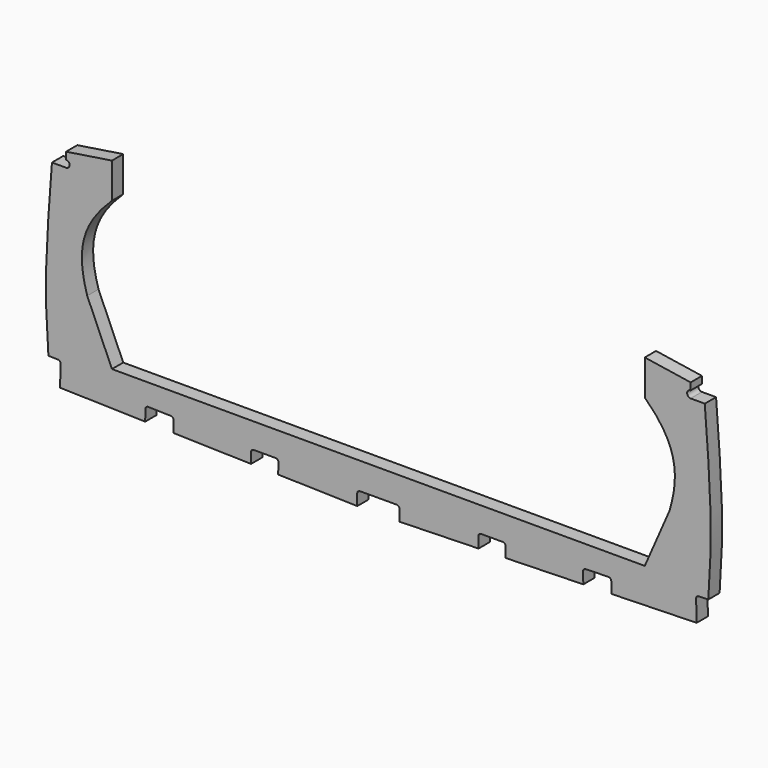
from build123d import *

# Parameters (mm, degrees)
F1_DEPTH = 25.4


with BuildPart() as f1:
    # F0 (on Front) → F1 (new body)
    with BuildSketch(Plane.XZ):
        with BuildLine():
            Line((-180.280449281, -69.793186067), (-37.9985533655, -73.516196597))
            Line((-37.9985533655, -73.516196597), (-37.9985533655, -53.3922091126))
            ThreePointArc((-37.9985533655, -53.3922091126), (-36.3574166334, -49.6531424612), (-32.4943724898, -48.3299496779))
            Line((-32.4943724898, -48.3299496779), (32.4792108915, -48.1490081299))
            ThreePointArc((32.4792108915, -48.1490081299), (36.3518127667, -49.4657614096), (37.9985533655, -53.209974262))
            Line((37.9985533655, -53.209974262), (37.9985533655, -73.516196597))
            Line((37.9985533655, -73.516196597), (180.280449281, -69.793186067))
            Line((180.280449281, -69.793186067), (179.7684819711, -50.3384282921))
            ThreePointArc((179.7684819711, -50.3384282921), (181.2076799987, -46.6602509384), (184.8467238815, -45.124790347))
            Line((184.8467238815, -45.124790347), (224.0474202454, -45.124790347))
            ThreePointArc((224.0474202454, -45.124790347), (227.6395226938, -46.6126878986), (229.1274202454, -50.204790347))
            Line((229.1274202454, -50.204790347), (229.1274202454, -68.8998913716))
            Line((229.1274202454, -68.8998913716), (368.779072779, -65.2248478839))
            Line((368.779072779, -65.2248478839), (368.2445209989, -44.9118802426))
            ThreePointArc((368.2445209989, -44.9118802426), (369.6374073208, -41.2818793035), (373.1891249642, -39.7000003873))
            Line((373.1891249642, -39.7000003873), (413.8150602467, -38.6308968272))
            ThreePointArc((413.8150602467, -38.6308968272), (417.4450611859, -40.0237831491), (419.0269401021, -43.5755007925))
            Line((419.0269401021, -43.5755007925), (419.5614918821, -63.8884684338))
            Line((419.5614918821, -63.8884684338), (572.7053844218, -59.8583659985))
            Line((572.7053844218, -59.8583659985), (571.7030998342, -21.7715516712))
            ThreePointArc((571.7030998342, -21.7715516712), (573.0959861561, -18.141550732), (576.6477037995, -16.5596718159))
            Line((576.6477037995, -16.5596718159), (593.6560001815, -16.112085069))
            add(Edge.make_bspline(
                [(593.6560001815, -16.112085069), (596.1080901801, 20.5341002257), (601.6949471336, 104.0289944805), (592.471101525, 224.502637459), (587.295632267, 292.1)],
                knots=[0, 0, 0, 0, 0.4389033081, 1, 1, 1, 1], degree=3))
            Line((587.295632267, 292.1), (561.895632267, 292.1))
            ThreePointArc((561.895632267, 292.1), (555.545632267, 298.45), (561.895632267, 304.8))
            Line((561.895632267, 304.8), (561.895632267, 317.5))
            Line((561.895632267, 317.5), (479.345632267, 330.2))
            Line((479.345632267, 330.2), (479.345632267, 266.595095396))
            add(Edge.make_bspline(
                [(479.345632267, 266.595095396), (537.2284650803, 211.8650227785), (542.5910949707, 164.6739989519), (523.795632267, 101.6)],
                knots=[0, 0, 0, 0, 170.8776872642, 170.8776872642, 170.8776872642, 170.8776872642], degree=3))
            Line((523.795632267, 101.6), (479.345632267, 0))
            Line((479.345632267, 0), (0, 0))
            Line((0, 0), (-479.345632267, 0))
            Line((-479.345632267, 0), (-523.795632267, 101.6))
            add(Edge.make_bspline(
                [(-479.345632267, 266.595095396), (-537.2284650803, 211.8650227785), (-542.5910949707, 164.6739989519), (-523.795632267, 101.6)],
                knots=[0, 0, 0, 0, 170.8776872642, 170.8776872642, 170.8776872642, 170.8776872642], degree=3))
            Line((-479.345632267, 266.595095396), (-479.345632267, 330.2))
            Line((-479.345632267, 330.2), (-561.895632267, 317.5))
            Line((-561.895632267, 317.5), (-561.895632267, 304.8))
            ThreePointArc((-561.895632267, 304.8), (-555.545632267, 298.45), (-561.895632267, 292.1))
            Line((-561.895632267, 292.1), (-587.295632267, 292.1))
            add(Edge.make_bspline(
                [(-593.6560001815, -16.112085069), (-596.1080901801, 20.5341002257), (-601.6949471336, 104.0289944805), (-592.471101525, 224.502637459), (-587.295632267, 292.1)],
                knots=[0, 0, 0, 0, 0.4389033081, 1, 1, 1, 1], degree=3))
            Line((-593.6560001815, -16.112085069), (-576.6477037995, -16.5596718159))
            ThreePointArc((-576.6477037995, -16.5596718159), (-573.0959861561, -18.141550732), (-571.7030998342, -21.7715516712))
            Line((-571.7030998342, -21.7715516712), (-572.7053844218, -59.8583659985))
            Line((-572.7053844218, -59.8583659985), (-419.5614918821, -63.8884684338))
            Line((-419.5614918821, -63.8884684338), (-419.0269401021, -43.5755007925))
            ThreePointArc((-419.0269401021, -43.5755007925), (-417.4450611859, -40.0237831491), (-413.8150602467, -38.6308968272))
            Line((-413.8150602467, -38.6308968272), (-373.1891249642, -39.7000003873))
            ThreePointArc((-373.1891249642, -39.7000003873), (-369.6374073208, -41.2818793035), (-368.2445209989, -44.9118802426))
            Line((-368.2445209989, -44.9118802426), (-368.779072779, -65.2248478839))
            Line((-368.779072779, -65.2248478839), (-229.1274202454, -68.8998913716))
            Line((-229.1274202454, -68.8998913716), (-229.1274202454, -50.204790347))
            ThreePointArc((-229.1274202454, -50.204790347), (-227.6395226938, -46.6126878986), (-224.0474202454, -45.124790347))
            Line((-224.0474202454, -45.124790347), (-184.8467238815, -45.124790347))
            ThreePointArc((-184.8467238815, -45.124790347), (-181.2076799987, -46.6602509384), (-179.7684819711, -50.3384282921))
            Line((-179.7684819711, -50.3384282921), (-180.280449281, -69.793186067))
        make_face()
    extrude(amount=F1_DEPTH)


solid = f1.part
